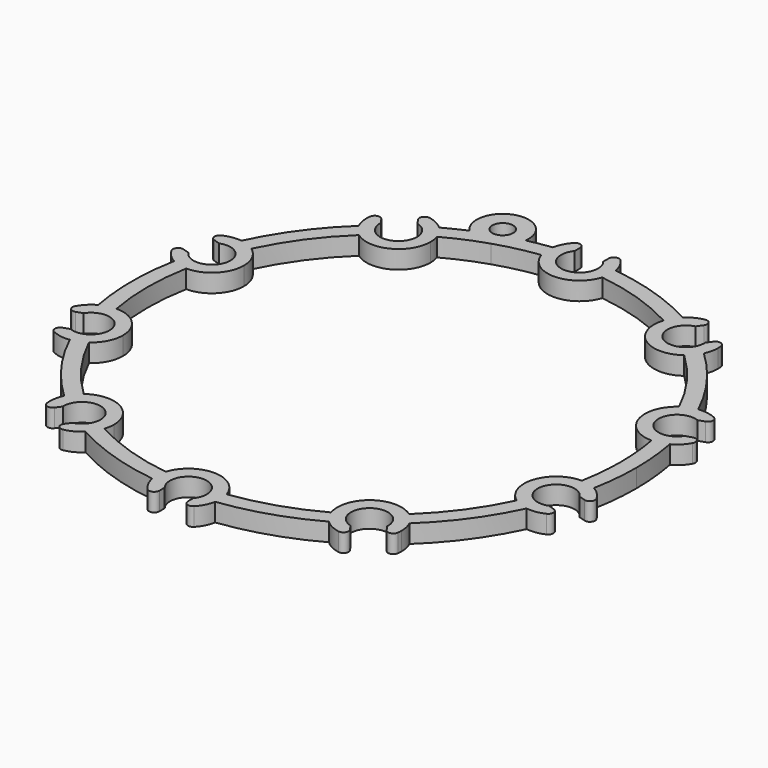
from build123d import *

# Parameters (mm, degrees)
F1_DEPTH = 3.5
F2_R     = 2
F3_DEPTH = 25
F4_R     = 1


with BuildPart() as f1:
    # F0 (on Top) → F1 (new body)
    with BuildSketch(Plane.XY):
        with BuildLine():
            ThreePointArc((5.8561077123, 45.1215691489), (6.0760827196, 46.0493587508), (6.15, 47))
            ThreePointArc((6.15, 47), (6.1241621044, 47.5631505297), (6.0468655222, 48.1215691489))
            ThreePointArc((6.0468655222, 48.1215691489), (0, 48.5), (-6.0468655222, 48.1215691489))
            ThreePointArc((-6.0468655222, 48.1215691489), (-6.1376048224, 46.6097346485), (-5.8561077123, 45.1215691489))
            ThreePointArc((-5.8561077123, 45.1215691489), (0, 45.5), (5.8561077123, 45.1215691489))
        make_face()
        with BuildLine():
            ThreePointArc((6.0468655222, 48.1215691489), (6.1241621044, 47.5631505297), (6.15, 47))
            ThreePointArc((6.15, 47), (6.0760827196, 46.0493587508), (5.8561077123, 45.1215691489))
            ThreePointArc((5.8561077123, 45.1215691489), (14.0602732441, 43.2730714914), (21.7841022459, 39.9462500035))
            ThreePointArc((21.7841022459, 39.9462500035), (22.4310880336, 41.315661033), (23.3931316927, 42.4854256141))
            ThreePointArc((23.3931316927, 42.4854256141), (14.9873242272, 46.1262410403), (6.0468655222, 48.1215691489))
        make_face()
        with BuildLine():
            ThreePointArc((-6.0468655222, 48.1215691489), (0, 48.5), (6.0468655222, 48.1215691489))
            ThreePointArc((6.0468655222, 48.1215691489), (0, 53.15), (-6.0468655222, 48.1215691489))
        make_face()
        with BuildLine():
            ThreePointArc((-5.8561077123, 45.1215691489), (0, 40.85), (5.8561077123, 45.1215691489))
            ThreePointArc((5.8561077123, 45.1215691489), (0, 45.5), (-5.8561077123, 45.1215691489))
        make_face()
        with BuildLine():
            ThreePointArc((-5.8561077123, 45.1215691489), (-6.1376048224, 46.6097346485), (-6.0468655222, 48.1215691489))
            ThreePointArc((-6.0468655222, 48.1215691489), (-8.3614389621, 47.7738038938), (-10.6565393192, 47.3147774986))
            ThreePointArc((-10.6565393192, 47.3147774986), (-11.7808917587, 44.8075690262), (-14.0602732607, 43.273071486))
            ThreePointArc((-14.0602732607, 43.273071486), (-10.0009896344, 44.3872752749), (-5.8561077123, 45.1215691489))
        make_face()
        with BuildLine():
            ThreePointArc((33.1771656331, 35.3769088609), (28.5075847362, 39.2373242272), (23.3931316927, 42.4854256141))
            ThreePointArc((23.3931316927, 42.4854256141), (22.4310880336, 41.315661033), (21.7841022459, 39.9462500035))
            ThreePointArc((21.7841022459, 39.9462500035), (26.7442289793, 36.8102732441), (31.2594835662, 33.0619825052))
            ThreePointArc((31.2594835662, 33.0619825052), (32.3619412457, 34.100473835), (33.1771656331, 35.3769088609))
        make_face()
        with BuildLine():
            ThreePointArc((33.7759068577, 38.0237987356), (30.0539650052, 43.6741999278), (23.3931316927, 42.4854256141))
            ThreePointArc((23.3931316927, 42.4854256141), (28.5075847362, 39.2373242272), (33.1771656331, 35.3769088609))
            ThreePointArc((33.1771656331, 35.3769088609), (33.624354218, 36.66691655), (33.7759068577, 38.0237987356))
        make_face()
        with BuildLine():
            ThreePointArc((31.2594835662, 33.0619825052), (26.7442289793, 36.8102732441), (21.7841022459, 39.9462500035))
            ThreePointArc((21.7841022459, 39.9462500035), (24.0110275561, 33.0483442202), (31.2594835662, 33.0619825052))
        make_face()
        with BuildLine():
            ThreePointArc((-14.0602732607, 43.273071486), (-11.7808917587, 44.8075690262), (-10.6565393192, 47.3147774986))
            ThreePointArc((-10.6565393192, 47.3147774986), (-14.9873242272, 46.1262410403), (-19.1896070187, 44.5422157337))
            ThreePointArc((-19.1896070187, 44.5422157337), (-16.8062866399, 43.1747192576), (-14.0602732607, 43.273071486))
        make_face()
        with BuildLine():
            ThreePointArc((-19.1896070187, 44.5422157337), (-14.9873242272, 46.1262410403), (-10.6565393192, 47.3147774986))
            ThreePointArc((-10.6565393192, 47.3147774986), (-10.6181699057, 47.670649225), (-10.6053582159, 48.0283540729))
            ThreePointArc((-10.6053582159, 48.0283540729), (-17.4866816844, 52.6609151364), (-19.1896070187, 44.5422157337))
        make_face()
        with BuildLine():
            ThreePointArc((43.8977477044, 20.6212935211), (39.2373242272, 28.5075847362), (33.1771656331, 35.3769088609))
            ThreePointArc((33.1771656331, 35.3769088609), (32.3619412457, 34.100473835), (31.2594835662, 33.0619825052))
            ThreePointArc((31.2594835662, 33.0619825052), (36.8102732441, 26.7442289793), (41.1035255606, 19.5128210798))
            ThreePointArc((41.1035255606, 19.5128210798), (42.4318676654, 20.2404091705), (43.8977477044, 20.6212935211))
        make_face()
        with BuildLine():
            ThreePointArc((-21.7841022459, 39.9462500035), (-17.9992152373, 41.7884942399), (-14.0602732607, 43.273071486))
            ThreePointArc((-14.0602732607, 43.273071486), (-16.8062866399, 43.1747192576), (-19.1896070187, 44.5422157337))
            ThreePointArc((-19.1896070187, 44.5422157337), (-21.316191157, 43.5645497459), (-23.3931316927, 42.4854256141))
            ThreePointArc((-23.3931316927, 42.4854256141), (-22.4310880336, 41.315661033), (-21.7841022459, 39.9462500035))
        make_face()
        with BuildLine():
            ThreePointArc((47.6349161225, 9.1194718049), (46.1262410403, 14.9873242272), (43.8977477044, 20.6212935211))
            ThreePointArc((43.8977477044, 20.6212935211), (42.4318676654, 20.2404091705), (41.1035255606, 19.5128210798))
            ThreePointArc((41.1035255606, 19.5128210798), (43.2730714914, 14.0602732441), (44.7227991685, 8.37384228))
            ThreePointArc((44.7227991685, 8.37384228), (46.2251160551, 8.565991049), (47.6349161225, 9.1194718049))
        make_face()
        with BuildLine():
            ThreePointArc((50.8496562659, 14.5237987356), (48.7549467824, 19.1473383782), (43.8977477044, 20.6212935211))
            ThreePointArc((43.8977477044, 20.6212935211), (46.1262410403, 14.9873242272), (47.6349161225, 9.1194718049))
            ThreePointArc((47.6349161225, 9.1194718049), (49.9852190608, 11.3797049169), (50.8496562659, 14.5237987356))
        make_face()
        with BuildLine():
            ThreePointArc((-31.2594835662, 33.0619825052), (-26.7442289793, 36.8102732441), (-21.7841022459, 39.9462500035))
            ThreePointArc((-21.7841022459, 39.9462500035), (-22.4310880336, 41.315661033), (-23.3931316927, 42.4854256141))
            ThreePointArc((-23.3931316927, 42.4854256141), (-28.5075847362, 39.2373242272), (-33.1771656331, 35.3769088609))
            ThreePointArc((-33.1771656331, 35.3769088609), (-32.3619412457, 34.100473835), (-31.2594835662, 33.0619825052))
        make_face()
        with BuildLine():
            ThreePointArc((-21.4759068577, 38.0237987356), (-21.5534444922, 38.9972980005), (-21.7841022459, 39.9462500035))
            ThreePointArc((-21.7841022459, 39.9462500035), (-26.7442289793, 36.8102732441), (-31.2594835662, 33.0619825052))
            ThreePointArc((-31.2594835662, 33.0619825052), (-24.8441804834, 32.5388649732), (-21.4759068577, 38.0237987356))
        make_face()
        with BuildLine():
            ThreePointArc((44.7227991685, 8.37384228), (43.2730714914, 14.0602732441), (41.1035255606, 19.5128210798))
            ThreePointArc((41.1035255606, 19.5128210798), (38.8506586907, 12.6233442202), (44.7227991685, 8.37384228))
        make_face()
        with BuildLine():
            ThreePointArc((-33.1771656331, 35.3769088609), (-28.5075847362, 39.2373242272), (-23.3931316927, 42.4854256141))
            ThreePointArc((-23.3931316927, 42.4854256141), (-31.2407861593, 42.999253251), (-33.1771656331, 35.3769088609))
        make_face()
        with BuildLine():
            ThreePointArc((48.5, 0), (48.2832446711, 4.5802056754), (47.6349161225, 9.1194718049))
            ThreePointArc((47.6349161225, 9.1194718049), (46.2251160551, 8.565991049), (44.7227991685, 8.37384228))
            ThreePointArc((44.7227991685, 8.37384228), (45.3052831476, 4.2049160415), (45.5, 0))
            ThreePointArc((45.5, 0), (45.3052831476, -4.2049160415), (44.7227991685, -8.37384228))
            ThreePointArc((44.7227991685, -8.37384228), (46.2251160551, -8.565991049), (47.6349161225, -9.1194718049))
            ThreePointArc((47.6349161225, -9.1194718049), (48.2832446711, -4.5802056754), (48.5, 0))
        make_face()
        with BuildLine():
            ThreePointArc((-41.1035255606, 19.5128210798), (-36.8102732441, 26.7442289793), (-31.2594835662, 33.0619825052))
            ThreePointArc((-31.2594835662, 33.0619825052), (-32.3619412457, 34.100473835), (-33.1771656331, 35.3769088609))
            ThreePointArc((-33.1771656331, 35.3769088609), (-39.2373242272, 28.5075847362), (-43.8977477044, 20.6212935211))
            ThreePointArc((-43.8977477044, 20.6212935211), (-42.4318676654, 20.2404091705), (-41.1035255606, 19.5128210798))
        make_face()
        with BuildLine():
            ThreePointArc((-44.7227991685, 8.37384228), (-43.2730714914, 14.0602732441), (-41.1035255606, 19.5128210798))
            ThreePointArc((-41.1035255606, 19.5128210798), (-42.4318676654, 20.2404091705), (-43.8977477044, 20.6212935211))
            ThreePointArc((-43.8977477044, 20.6212935211), (-46.1262410403, 14.9873242272), (-47.6349161225, 9.1194718049))
            ThreePointArc((-47.6349161225, 9.1194718049), (-46.2251160551, 8.565991049), (-44.7227991685, 8.37384228))
        make_face()
        with BuildLine():
            ThreePointArc((-38.5496562659, 14.5237987356), (-39.22522918, 17.3261456237), (-41.1035255606, 19.5128210798))
            ThreePointArc((-41.1035255606, 19.5128210798), (-43.2730714914, 14.0602732441), (-44.7227991685, 8.37384228))
            ThreePointArc((-44.7227991685, 8.37384228), (-40.3591395254, 10.1669174628), (-38.5496562659, 14.5237987356))
        make_face()
        with BuildLine():
            ThreePointArc((-47.6349161225, 9.1194718049), (-46.1262410403, 14.9873242272), (-43.8977477044, 20.6212935211))
            ThreePointArc((-43.8977477044, 20.6212935211), (-50.5486538411, 16.424253251), (-47.6349161225, 9.1194718049))
        make_face()
        with BuildLine():
            ThreePointArc((43.8977477044, -20.6212935211), (46.1262410403, -14.9873242272), (47.6349161225, -9.1194718049))
            ThreePointArc((47.6349161225, -9.1194718049), (46.2251160551, -8.565991049), (44.7227991685, -8.37384228))
            ThreePointArc((44.7227991685, -8.37384228), (43.2730714914, -14.0602732441), (41.1035255606, -19.5128210798))
            ThreePointArc((41.1035255606, -19.5128210798), (42.4318676654, -20.2404091705), (43.8977477044, -20.6212935211))
        make_face()
        with BuildLine():
            ThreePointArc((50.8496562659, -14.5237987356), (49.9852190608, -11.3797049169), (47.6349161225, -9.1194718049))
            ThreePointArc((47.6349161225, -9.1194718049), (46.1262410403, -14.9873242272), (43.8977477044, -20.6212935211))
            ThreePointArc((43.8977477044, -20.6212935211), (48.7549467824, -19.1473383782), (50.8496562659, -14.5237987356))
        make_face()
        with BuildLine():
            ThreePointArc((-44.7227991685, -8.37384228), (-45.5, 0), (-44.7227991685, 8.37384228))
            ThreePointArc((-44.7227991685, 8.37384228), (-46.2251160551, 8.565991049), (-47.6349161225, 9.1194718049))
            ThreePointArc((-47.6349161225, 9.1194718049), (-48.5, 0), (-47.6349161225, -9.1194718049))
            ThreePointArc((-47.6349161225, -9.1194718049), (-46.2251160551, -8.565991049), (-44.7227991685, -8.37384228))
        make_face()
        with BuildLine():
            ThreePointArc((41.1035255606, -19.5128210798), (43.2730714914, -14.0602732441), (44.7227991685, -8.37384228))
            ThreePointArc((44.7227991685, -8.37384228), (38.8506586907, -12.6233442202), (41.1035255606, -19.5128210798))
        make_face()
        with BuildLine():
            ThreePointArc((33.1771656331, -35.3769088609), (39.2373242272, -28.5075847362), (43.8977477044, -20.6212935211))
            ThreePointArc((43.8977477044, -20.6212935211), (42.4318676654, -20.2404091705), (41.1035255606, -19.5128210798))
            ThreePointArc((41.1035255606, -19.5128210798), (36.8102732441, -26.7442289793), (31.2594835662, -33.0619825052))
            ThreePointArc((31.2594835662, -33.0619825052), (32.3619412457, -34.100473835), (33.1771656331, -35.3769088609))
        make_face()
        with BuildLine():
            ThreePointArc((-41.1035255606, -19.5128210798), (-43.2730714914, -14.0602732441), (-44.7227991685, -8.37384228))
            ThreePointArc((-44.7227991685, -8.37384228), (-46.2251160551, -8.565991049), (-47.6349161225, -9.1194718049))
            ThreePointArc((-47.6349161225, -9.1194718049), (-46.1262410403, -14.9873242272), (-43.8977477044, -20.6212935211))
            ThreePointArc((-43.8977477044, -20.6212935211), (-42.4318676654, -20.2404091705), (-41.1035255606, -19.5128210798))
        make_face()
        with BuildLine():
            ThreePointArc((-38.5496562659, -14.5237987356), (-40.3591395254, -10.1669174628), (-44.7227991685, -8.37384228))
            ThreePointArc((-44.7227991685, -8.37384228), (-43.2730714914, -14.0602732441), (-41.1035255606, -19.5128210798))
            ThreePointArc((-41.1035255606, -19.5128210798), (-39.22522918, -17.3261456237), (-38.5496562659, -14.5237987356))
        make_face()
        with BuildLine():
            ThreePointArc((-43.8977477044, -20.6212935211), (-46.1262410403, -14.9873242272), (-47.6349161225, -9.1194718049))
            ThreePointArc((-47.6349161225, -9.1194718049), (-50.5486538411, -16.424253251), (-43.8977477044, -20.6212935211))
        make_face()
        with BuildLine():
            ThreePointArc((23.3931316927, -42.4854256141), (28.5075847362, -39.2373242272), (33.1771656331, -35.3769088609))
            ThreePointArc((33.1771656331, -35.3769088609), (32.3619412457, -34.100473835), (31.2594835662, -33.0619825052))
            ThreePointArc((31.2594835662, -33.0619825052), (26.7442289793, -36.8102732441), (21.7841022459, -39.9462500035))
            ThreePointArc((21.7841022459, -39.9462500035), (22.4310880336, -41.315661033), (23.3931316927, -42.4854256141))
        make_face()
        with BuildLine():
            ThreePointArc((33.7759068577, -38.0237987356), (33.624354218, -36.66691655), (33.1771656331, -35.3769088609))
            ThreePointArc((33.1771656331, -35.3769088609), (28.5075847362, -39.2373242272), (23.3931316927, -42.4854256141))
            ThreePointArc((23.3931316927, -42.4854256141), (30.0539650052, -43.6741999278), (33.7759068577, -38.0237987356))
        make_face()
        with BuildLine():
            ThreePointArc((-31.2594835662, -33.0619825052), (-36.8102732441, -26.7442289793), (-41.1035255606, -19.5128210798))
            ThreePointArc((-41.1035255606, -19.5128210798), (-42.4318676654, -20.2404091705), (-43.8977477044, -20.6212935211))
            ThreePointArc((-43.8977477044, -20.6212935211), (-39.2373242272, -28.5075847362), (-33.1771656331, -35.3769088609))
            ThreePointArc((-33.1771656331, -35.3769088609), (-32.3619412457, -34.100473835), (-31.2594835662, -33.0619825052))
        make_face()
        with BuildLine():
            ThreePointArc((21.7841022459, -39.9462500035), (26.7442289793, -36.8102732441), (31.2594835662, -33.0619825052))
            ThreePointArc((31.2594835662, -33.0619825052), (24.0110275561, -33.0483442202), (21.7841022459, -39.9462500035))
        make_face()
        with BuildLine():
            ThreePointArc((6.0468655222, -48.1215691489), (14.9873242272, -46.1262410403), (23.3931316927, -42.4854256141))
            ThreePointArc((23.3931316927, -42.4854256141), (22.4310880336, -41.315661033), (21.7841022459, -39.9462500035))
            ThreePointArc((21.7841022459, -39.9462500035), (14.0602732441, -43.2730714914), (5.8561077123, -45.1215691489))
            ThreePointArc((5.8561077123, -45.1215691489), (6.0760827196, -46.0493587508), (6.15, -47))
            ThreePointArc((6.15, -47), (6.1241621044, -47.5631505297), (6.0468655222, -48.1215691489))
        make_face()
        with BuildLine():
            ThreePointArc((-21.7841022459, -39.9462500035), (-26.7442289793, -36.8102732441), (-31.2594835662, -33.0619825052))
            ThreePointArc((-31.2594835662, -33.0619825052), (-32.3619412457, -34.100473835), (-33.1771656331, -35.3769088609))
            ThreePointArc((-33.1771656331, -35.3769088609), (-28.5075847362, -39.2373242272), (-23.3931316927, -42.4854256141))
            ThreePointArc((-23.3931316927, -42.4854256141), (-22.4310880336, -41.315661033), (-21.7841022459, -39.9462500035))
        make_face()
        with BuildLine():
            ThreePointArc((-21.4759068577, -38.0237987356), (-24.8441804834, -32.5388649732), (-31.2594835662, -33.0619825052))
            ThreePointArc((-31.2594835662, -33.0619825052), (-26.7442289793, -36.8102732441), (-21.7841022459, -39.9462500035))
            ThreePointArc((-21.7841022459, -39.9462500035), (-21.5534444922, -38.9972980005), (-21.4759068577, -38.0237987356))
        make_face()
        with BuildLine():
            ThreePointArc((-23.3931316927, -42.4854256141), (-28.5075847362, -39.2373242272), (-33.1771656331, -35.3769088609))
            ThreePointArc((-33.1771656331, -35.3769088609), (-31.2407861593, -42.999253251), (-23.3931316927, -42.4854256141))
        make_face()
        with BuildLine():
            ThreePointArc((-6.0468655222, -48.1215691489), (0, -48.5), (6.0468655222, -48.1215691489))
            ThreePointArc((6.0468655222, -48.1215691489), (6.1241621044, -47.5631505297), (6.15, -47))
            ThreePointArc((6.15, -47), (6.0760827196, -46.0493587508), (5.8561077123, -45.1215691489))
            ThreePointArc((5.8561077123, -45.1215691489), (0, -45.5), (-5.8561077123, -45.1215691489))
            ThreePointArc((-5.8561077123, -45.1215691489), (-6.1376048224, -46.6097346485), (-6.0468655222, -48.1215691489))
        make_face()
        with BuildLine():
            ThreePointArc((-6.0468655222, -48.1215691489), (0, -53.15), (6.0468655222, -48.1215691489))
            ThreePointArc((6.0468655222, -48.1215691489), (0, -48.5), (-6.0468655222, -48.1215691489))
        make_face()
        with BuildLine():
            ThreePointArc((-5.8561077123, -45.1215691489), (-14.0602732441, -43.2730714914), (-21.7841022459, -39.9462500035))
            ThreePointArc((-21.7841022459, -39.9462500035), (-22.4310880336, -41.315661033), (-23.3931316927, -42.4854256141))
            ThreePointArc((-23.3931316927, -42.4854256141), (-14.9873242272, -46.1262410403), (-6.0468655222, -48.1215691489))
            ThreePointArc((-6.0468655222, -48.1215691489), (-6.1376048224, -46.6097346485), (-5.8561077123, -45.1215691489))
        make_face()
        with BuildLine():
            ThreePointArc((-5.8561077123, -45.1215691489), (0, -45.5), (5.8561077123, -45.1215691489))
            ThreePointArc((5.8561077123, -45.1215691489), (0, -40.85), (-5.8561077123, -45.1215691489))
        make_face()
    extrude(amount=F1_DEPTH)

    # F2 (on face) → F3 (cut)
    with BuildSketch(Plane.XY.offset(3.5)):
        with BuildLine():
            ThreePointArc((-2.75, 49.2449944321), (-1.1916375288, 43.6559754786), (3.55, 47))
            ThreePointArc((3.55, 47), (3.3440245214, 48.1916375288), (2.75, 49.2449944321))
            Line((2.75, 49.2449944321), (2.75, 47.0036193728))
            Line((2.75, 47.0036193728), (-2.75, 47.0036193728))
            Line((-2.75, 47.0036193728), (-2.75, 49.2449944321))
        make_face()
        with BuildLine():
            Line((2.75, 47.0036193728), (2.75, 49.2449944321))
            ThreePointArc((2.75, 49.2449944321), (0, 50.55), (-2.75, 49.2449944321))
            Line((-2.75, 49.2449944321), (-2.75, 47.0036193728))
            Line((-2.75, 47.0036193728), (2.75, 47.0036193728))
        make_face()
        with BuildLine():
            ThreePointArc((-2.75, 49.2449944321), (0, 50.55), (2.75, 49.2449944321))
            Line((2.75, 49.2449944321), (2.75, 59.4616867602))
            Line((2.75, 59.4616867602), (-2.75, 59.4616867602))
            Line((-2.75, 59.4616867602), (-2.75, 49.2449944321))
        make_face()
        with BuildLine():
            ThreePointArc((-31.1702782109, 38.2236279396), (-27.7258610878, 34.4752061763), (-24.0759068577, 38.0237987356))
            ThreePointArc((-24.0759068577, 38.0237987356), (-24.8137867935, 40.1904737792), (-26.7206847419, 41.4564468272))
            ThreePointArc((-26.7206847419, 41.4564468272), (-29.7125445034, 40.8958090657), (-31.1702782109, 38.2236279396))
        make_face()
        with BuildLine():
            ThreePointArc((-31.1702782109, 38.2236279396), (-29.7125445034, 40.8958090657), (-26.7206847419, 41.4564468272))
            Line((-26.7206847419, 41.4564468272), (-32.7259058195, 49.721924547))
            Line((-32.7259058195, 49.721924547), (-37.1754992886, 46.4891056594))
            Line((-37.1754992886, 46.4891056594), (-31.1702782109, 38.2236279396))
        make_face()
        with BuildLine():
            ThreePointArc((-47.6845695841, 12.6021347476), (-43.6981429808, 11.1179991027), (-41.1496562659, 14.5237987356))
            ThreePointArc((-41.1496562659, 14.5237987356), (-42.6947105639, 17.4534220445), (-45.984976115, 17.8329455872))
            ThreePointArc((-45.984976115, 17.8329455872), (-48.0759068987, 15.6208090657), (-47.6845695841, 12.6021347476))
        make_face()
        with BuildLine():
            ThreePointArc((-47.6845695841, 12.6021347476), (-48.0759068987, 15.6208090657), (-45.984976115, 17.8329455872))
            Line((-45.984976115, 17.8329455872), (-55.7016279286, 20.9900771429))
            Line((-55.7016279286, 20.9900771429), (-57.4012213977, 15.7592663033))
            Line((-57.4012213977, 15.7592663033), (-47.6845695841, 12.6021347476))
        make_face()
        with BuildLine():
            ThreePointArc((-45.984976115, -17.8329455872), (-42.6947105639, -17.4534220445), (-41.1496562659, -14.5237987356))
            ThreePointArc((-41.1496562659, -14.5237987356), (-43.6981429808, -11.1179991027), (-47.6845695841, -12.6021347476))
            ThreePointArc((-47.6845695841, -12.6021347476), (-48.0759068987, -15.6208090657), (-45.984976115, -17.8329455872))
        make_face()
        with BuildLine():
            ThreePointArc((-45.984976115, -17.8329455872), (-48.0759068987, -15.6208090657), (-47.6845695841, -12.6021347476))
            Line((-47.6845695841, -12.6021347476), (-57.4012213977, -15.7592663033))
            Line((-57.4012213977, -15.7592663033), (-55.7016279286, -20.9900771429))
            Line((-55.7016279286, -20.9900771429), (-45.984976115, -17.8329455872))
        make_face()
        with BuildLine():
            ThreePointArc((-26.7206847419, -41.4564468272), (-24.8137867935, -40.1904737792), (-24.0759068577, -38.0237987356))
            ThreePointArc((-24.0759068577, -38.0237987356), (-27.7258610878, -34.4752061763), (-31.1702782109, -38.2236279396))
            ThreePointArc((-31.1702782109, -38.2236279396), (-29.7125445034, -40.8958090657), (-26.7206847419, -41.4564468272))
        make_face()
        with BuildLine():
            ThreePointArc((-26.7206847419, -41.4564468272), (-29.7125445034, -40.8958090657), (-31.1702782109, -38.2236279396))
            Line((-31.1702782109, -38.2236279396), (-37.1754992886, -46.4891056594))
            Line((-37.1754992886, -46.4891056594), (-32.7259058195, -49.721924547))
            Line((-32.7259058195, -49.721924547), (-26.7206847419, -41.4564468272))
        make_face()
        with BuildLine():
            ThreePointArc((2.75, -49.2449944321), (3.3440245214, -48.1916375288), (3.55, -47))
            ThreePointArc((3.55, -47), (-1.1916375288, -43.6559754786), (-2.75, -49.2449944321))
            ThreePointArc((-2.75, -49.2449944321), (0, -50.55), (2.75, -49.2449944321))
        make_face()
        with BuildLine():
            ThreePointArc((2.75, -49.2449944321), (0, -50.55), (-2.75, -49.2449944321))
            Line((-2.75, -49.2449944321), (-2.75, -59.4616867602))
            Line((-2.75, -59.4616867602), (2.75, -59.4616867602))
            Line((2.75, -59.4616867602), (2.75, -49.2449944321))
        make_face()
        with BuildLine():
            ThreePointArc((31.1702782109, -38.2236279396), (31.174499417, -38.1237529657), (31.1759068577, -38.0237987356))
            ThreePointArc((31.1759068577, -38.0237987356), (25.4592318142, -35.2116786714), (26.7206847419, -41.4564468272))
            ThreePointArc((26.7206847419, -41.4564468272), (29.7125445034, -40.8958090657), (31.1702782109, -38.2236279396))
        make_face()
        with BuildLine():
            ThreePointArc((31.1702782109, -38.2236279396), (29.7125445034, -40.8958090657), (26.7206847419, -41.4564468272))
            Line((26.7206847419, -41.4564468272), (32.7259058195, -49.721924547))
            Line((32.7259058195, -49.721924547), (37.1754992886, -46.4891056594))
            Line((37.1754992886, -46.4891056594), (31.1702782109, -38.2236279396))
        make_face()
        with BuildLine():
            ThreePointArc((45.984976115, -17.8329455872), (47.6292795748, -16.5287444376), (48.2496562659, -14.5237987356))
            ThreePointArc((48.2496562659, -14.5237987356), (48.1054558988, -13.5222854505), (47.6845695841, -12.6021347476))
            ThreePointArc((47.6845695841, -12.6021347476), (41.323405633, -13.4267884056), (45.984976115, -17.8329455872))
        make_face()
        with BuildLine():
            ThreePointArc((47.6845695841, -12.6021347476), (48.1054558988, -13.5222854505), (48.2496562659, -14.5237987356))
            ThreePointArc((48.2496562659, -14.5237987356), (47.6292795748, -16.5287444376), (45.984976115, -17.8329455872))
            Line((45.984976115, -17.8329455872), (55.7016279286, -20.9900771429))
            Line((55.7016279286, -20.9900771429), (57.4012213977, -15.7592663033))
            Line((57.4012213977, -15.7592663033), (47.6845695841, -12.6021347476))
        make_face()
        with BuildLine():
            ThreePointArc((47.6845695841, 12.6021347476), (48.1054558988, 13.5222854505), (48.2496562659, 14.5237987356))
            ThreePointArc((48.2496562659, 14.5237987356), (47.6292795748, 16.5287444376), (45.984976115, 17.8329455872))
            ThreePointArc((45.984976115, 17.8329455872), (41.323405633, 13.4267884056), (47.6845695841, 12.6021347476))
        make_face()
        with BuildLine():
            ThreePointArc((45.984976115, 17.8329455872), (47.6292795748, 16.5287444376), (48.2496562659, 14.5237987356))
            ThreePointArc((48.2496562659, 14.5237987356), (48.1054558988, 13.5222854505), (47.6845695841, 12.6021347476))
            Line((47.6845695841, 12.6021347476), (57.4012213977, 15.7592663033))
            Line((57.4012213977, 15.7592663033), (55.7016279286, 20.9900771429))
            Line((55.7016279286, 20.9900771429), (45.984976115, 17.8329455872))
        make_face()
        with BuildLine():
            ThreePointArc((26.7206847419, 41.4564468272), (25.4592318142, 35.2116786714), (31.1759068577, 38.0237987356))
            ThreePointArc((31.1759068577, 38.0237987356), (31.174499417, 38.1237529657), (31.1702782109, 38.2236279396))
            ThreePointArc((31.1702782109, 38.2236279396), (29.7125445034, 40.8958090657), (26.7206847419, 41.4564468272))
        make_face()
        with BuildLine():
            ThreePointArc((26.7206847419, 41.4564468272), (29.7125445034, 40.8958090657), (31.1702782109, 38.2236279396))
            Line((31.1702782109, 38.2236279396), (37.1754992886, 46.4891056594))
            Line((37.1754992886, 46.4891056594), (32.7259058195, 49.721924547))
            Line((32.7259058195, 49.721924547), (26.7206847419, 41.4564468272))
        make_face()
        with Locations((-15.6053582159, 48.0283540729)):
            Circle(F2_R)
    extrude(amount=-F3_DEPTH, mode=Mode.SUBTRACT)

    # F4
    f4_edges = [f1.edges().sort_by_distance(p)[0] for p in [
        (-49.081535, -18.839079, 1.75),
        (-50.781128, -13.608268, 1.75),
        (-33.084057, -40.857718, 1.75),
        (-28.634463, -44.090537, 1.75),
        (-2.75, -52.500909, 1.75),
        (2.75, -52.500909, 1.75),
        (-49.081535, 18.839079, 1.75),
        (-28.634463, 44.090537, 1.75),
        (2.75, 52.500909, 1.75),
        (28.634463, 44.090537, 1.75),
        (-50.781128, 13.608268, 1.75),
        (-33.084057, 40.857718, 1.75),
        (-2.75, 52.500909, 1.75),
        (33.084057, 40.857718, 1.75),
        (49.081535, 18.839079, 1.75),
        (50.781128, 13.608268, 1.75),
        (28.634463, -44.090537, 1.75),
        (33.084057, -40.857718, 1.75),
        (49.081535, -18.839079, 1.75),
        (50.781128, -13.608268, 1.75),
    ]]
    fillet(f4_edges, radius=F4_R)


solid = f1.part
